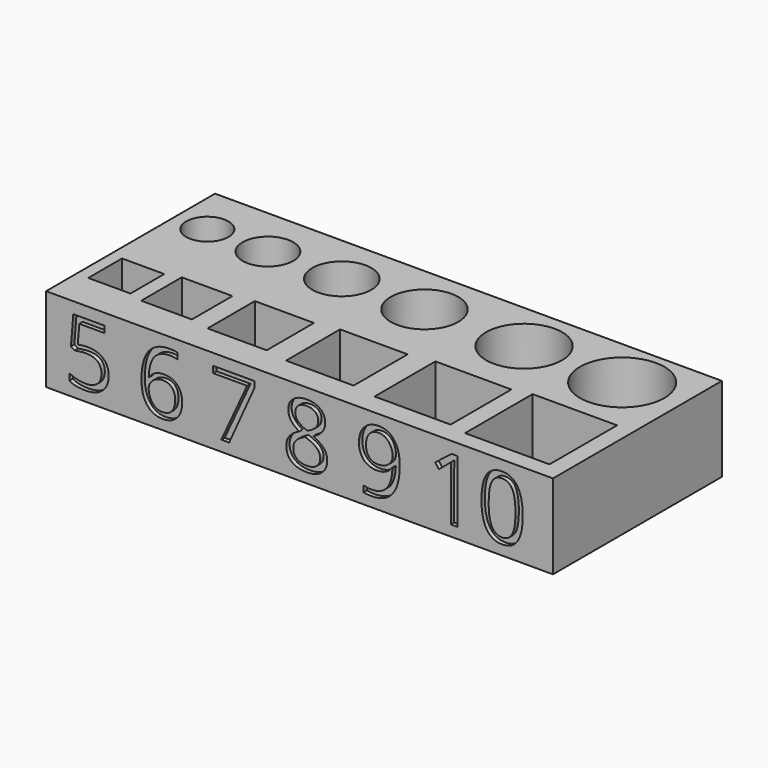
from build123d import *

# Parameters (mm, degrees)
F0_W         = 60
F0_H         = 25
F0_W_2       = 5
F0_H_2       = 5
F0_W_3       = 6
F0_H_3       = 6
F0_W_4       = 7
F0_H_4       = 7
F0_W_5       = 8
F0_H_5       = 8
F0_W_6       = 9
F0_H_6       = 9
F0_W_7       = 10
F0_H_7       = 10
F0_R         = 2.5
F0_R_2       = 3
F0_R_3       = 3.5
F0_R_4       = 4
F0_R_5       = 4.5
F0_R_6       = 5
F1_DEPTH     = 10
F2_TEXT_SIZE = 10.345334313
F3_DEPTH     = 0.5


# Not quite as in the source:
# - Text() gives the source's letters only with a copy of the font that has no kerning and outlines rounded to 1/6400 em; it was checked with that copy


with BuildPart() as f1:
    # F0 (on Top) → F1 (new body)
    with BuildSketch(Plane.XY):
        with Locations((0.4056511074, -0.2850802802)):
            Rectangle(F0_W, F0_H)
        with Locations((-25.7052196562, -5.7850802802)):
            Rectangle(F0_W_2, F0_H_2, mode=Mode.SUBTRACT)
        with Locations((-18.5344679654, -5.7850802802)):
            Rectangle(F0_W_3, F0_H_3, mode=Mode.SUBTRACT)
        with Locations((-9.7837172821, -5.7850802802)):
            Rectangle(F0_W_4, F0_H_4, mode=Mode.SUBTRACT)
        with Locations((0.4056511074, -5.7850802802)):
            Rectangle(F0_W_5, F0_H_5, mode=Mode.SUBTRACT)
        with Locations((11.7867002264, -5.7850802802)):
            Rectangle(F0_W_6, F0_H_6, mode=Mode.SUBTRACT)
        with Locations((23.3962056786, -5.7850802802)):
            Rectangle(F0_W_7, F0_H_7, mode=Mode.SUBTRACT)
        with Locations((-25.7052196562, 6.2149197198)):
            Circle(F0_R, mode=Mode.SUBTRACT)
        with Locations((-18.5344679654, 6.2149197198)):
            Circle(F0_R_2, mode=Mode.SUBTRACT)
        with Locations((-9.7837172821, 6.2149197198)):
            Circle(F0_R_3, mode=Mode.SUBTRACT)
        with Locations((0, 6.2149197198)):
            Circle(F0_R_4, mode=Mode.SUBTRACT)
        with Locations((11.7867002264, 6.2149197198)):
            Circle(F0_R_5, mode=Mode.SUBTRACT)
        with Locations((23.3962056786, 6.2149197198)):
            Circle(F0_R_6, mode=Mode.SUBTRACT)
    extrude(amount=F1_DEPTH)

    # F2 (on face) → F3 (cut)
    with BuildSketch(Plane.XZ.offset(12.7850802802)):
        with Locations((-27.5, 1.2677148799)):
            Text('5 6 7 8 9 10', F2_TEXT_SIZE, font='Open Sans', text_align=(TextAlign.LEFT, TextAlign.BOTTOM))
    extrude(amount=-F3_DEPTH, mode=Mode.SUBTRACT)


solid = f1.part
